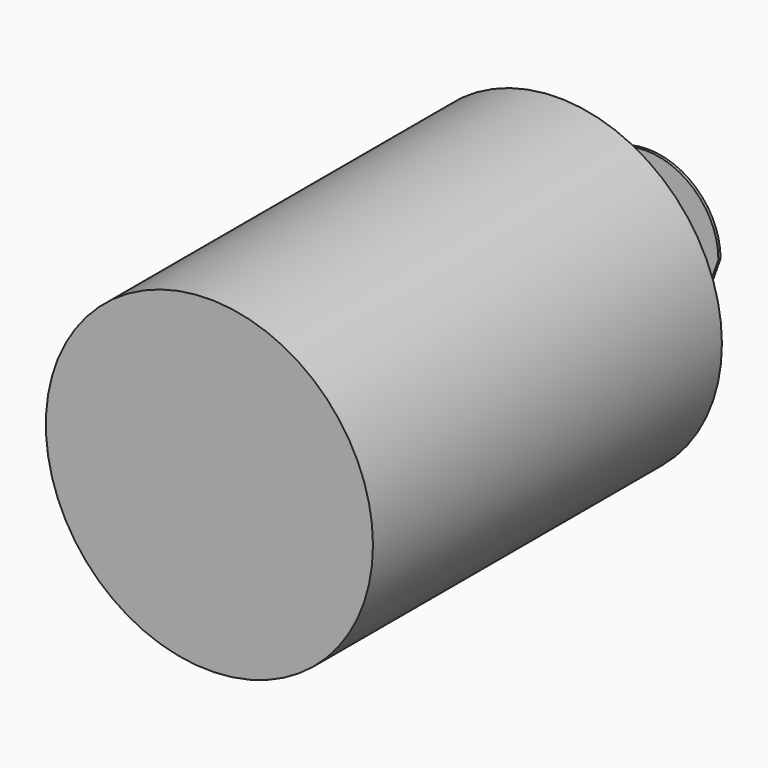
from build123d import *

# Parameters (mm, degrees)
F0_R     = 15
F1_DEPTH = 40
F2_R     = 1
F3_DEPTH = 10
F7_W     = 1.6538074706
F7_H     = 5.6983865798
F8_DEPTH = 0.25


# Not quite as in the source:
# - the program builds the solid bodies; features that only make, move or delete a surface that nothing else refers to are left out


with BuildPart() as f1:
    # F0 (on Front) → F1 (new body)
    with BuildSketch(Plane.XZ):
        Circle(F0_R)
    extrude(amount=F1_DEPTH)

    # F2 (on face) → F3 (join)
    with BuildSketch(Plane(origin=(0, 0, 0), x_dir=(-1, 0, 0), z_dir=(0, 1, 0))):
        Circle(F2_R)
    extrude(amount=F3_DEPTH)

    # F7 (on face) → F8 (join)
    with BuildSketch(Plane(origin=(0, 10, 0), x_dir=(-1, 0, 0), z_dir=(0, 1, 0))):
        with BuildLine():
            Line((2.032, -12.968), (6.6767431337, 0))
            ThreePointArc((6.6767431337, 0), (0, 6.6767431337), (-6.6767431337, 0))
            Line((-6.6767431337, 0), (-2.032, -12.968))
            Line((-2.032, -12.968), (2.032, -12.968))
        make_face()
        with Locations((0, -9.3933474272)):
            Rectangle(F7_W, F7_H, mode=Mode.SUBTRACT)
    extrude(amount=F8_DEPTH)


solid = f1.part
